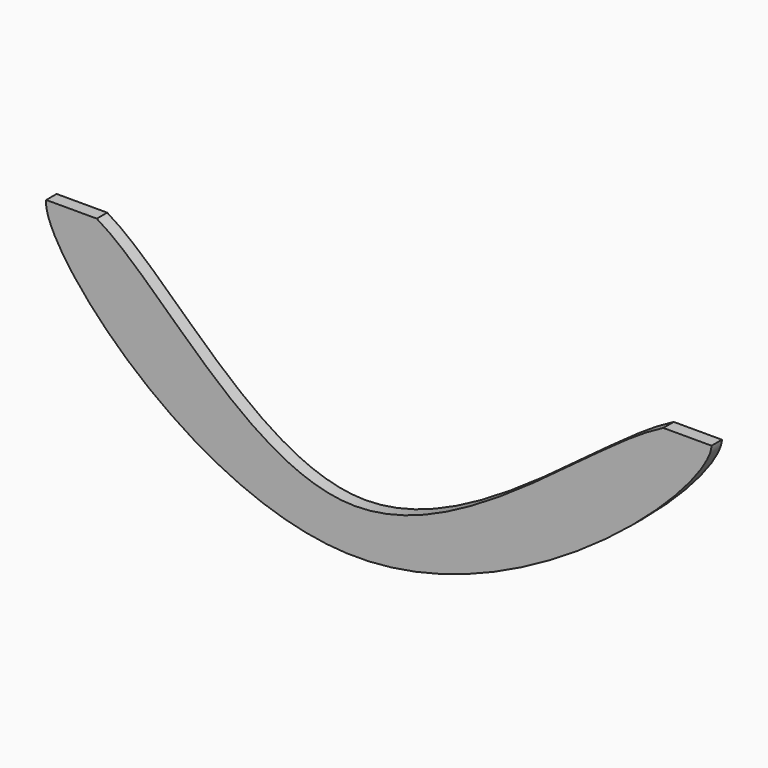
from build123d import *

# Parameters (mm, degrees)
F1_DEPTH = 1.27


with BuildPart() as f1:
    # F0 (on Front) → F1 (new body)
    with BuildSketch(Plane.XZ):
        with BuildLine():
            Line((-24.5671924204, 0), (-29.5004006475, 0))
            add(Edge.make_bspline(
                [(-29.5004006475, 0), (-29.9911045345, -4.2204110556), (-0.5226223556, -37.4558730435), (35.2213828045, -4.2021493862), (35.3921726346, 0)],
                knots=[0, 0, 0, 0, 0.2134826374, 0.44114243, 0.44114243, 0.44114243, 0.44114243], degree=3))
            Line((35.3921726346, 0), (30.6922141463, 0))
            add(Edge.make_bspline(
                [(30.6922141463, 0), (23.2773412139, -3.7026335354), (-0.7895870657, -29.3082281482), (-18.3109826379, -3.6709537273), (-24.5671924204, 0)],
                knots=[0.5181658423, 0.5181658423, 0.5181658423, 0.5181658423, 0.7278576819, 0.9210884694, 0.9210884694, 0.9210884694, 0.9210884694], degree=3))
        make_face()
    extrude(amount=F1_DEPTH)


solid = f1.part
